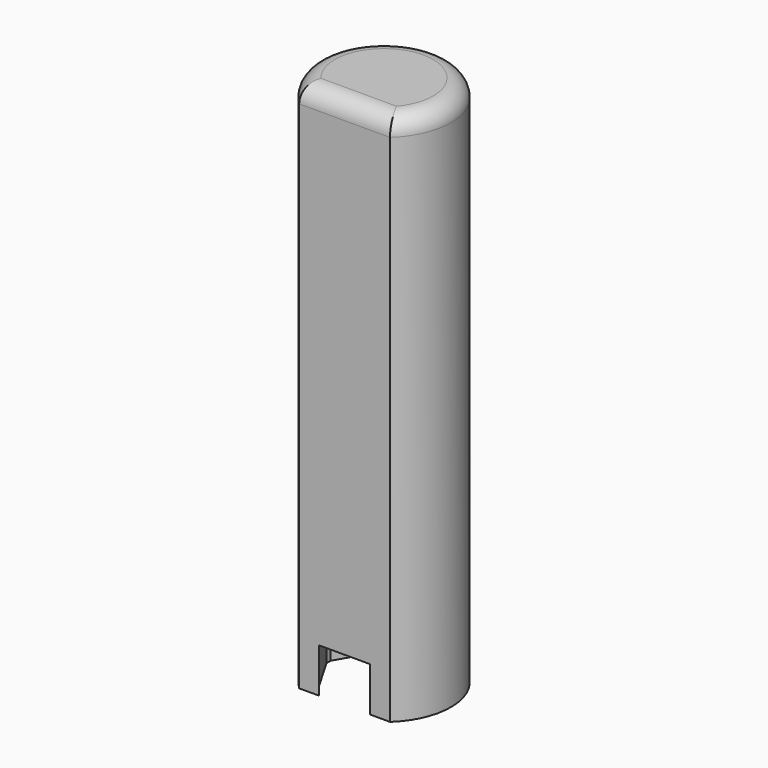
from build123d import *

# Parameters (mm, degrees)
F1_DEPTH    = 30
F2_DEPTH    = 2.5
F3_DEPTH    = 30
F4_T1_DEPTH = 10.1185935568
F4_T4_ANGLE = 350.8041938213


# Not quite as in the source:
# - a fillet or chamfer that OpenCascade refuses, or shapes differently, is made with other operations: its cross-section is extruded or revolved along the edge and cut away or added


with BuildPart() as f1:
    # F0 (on Top) → F1 (new body)
    with BuildSketch(Plane.XY):
        with BuildLine():
            Line((-1.4370107863, -2.775), (-1.602146997, -2.775))
            Line((-1.602146997, -2.775), (-2.5592967784, -2.775))
            ThreePointArc((-2.5592967784, -2.775), (0, -3.775), (2.5592967784, -2.775))
            Line((2.5592967784, -2.775), (1.602146997, -2.775))
            Line((1.602146997, -2.775), (1.4370107863, -2.775))
            ThreePointArc((1.4370107863, -2.775), (0, -3.125), (-1.4370107863, -2.775))
        make_face()
        with BuildLine():
            Line((-1.6847151023, 2.6319878465), (-1.602146997, 2.775))
            Line((-1.602146997, 2.775), (-1.4370107863, 2.775))
            ThreePointArc((-1.4370107863, 2.775), (0, 3.125), (1.4370107863, 2.775))
            Line((1.4370107863, 2.775), (1.602146997, 2.775))
            Line((1.602146997, 2.775), (1.6847151023, 2.6319878465))
            ThreePointArc((1.6847151023, 2.6319878465), (2.7063293868, 1.5625), (3.1217258887, 0.1430121535))
            Line((3.1217258887, 0.1430121535), (3.204293994, 0))
            Line((3.204293994, 0), (3.1217258887, -0.1430121535))
            ThreePointArc((3.1217258887, -0.1430121535), (2.7063293868, -1.5625), (1.6847151023, -2.6319878465))
            Line((1.6847151023, -2.6319878465), (1.602146997, -2.775))
            Line((1.602146997, -2.775), (2.5592967784, -2.775))
            ThreePointArc((2.5592967784, -2.775), (3.4577427853, -1.5148068625), (3.775, 0))
            ThreePointArc((3.775, 0), (-1.5148068625, 3.4577427853), (-2.5592967784, -2.775))
            Line((-2.5592967784, -2.775), (-1.602146997, -2.775))
            Line((-1.602146997, -2.775), (-1.6847151023, -2.6319878465))
            ThreePointArc((-1.6847151023, -2.6319878465), (-2.7063293868, -1.5625), (-3.1217258887, -0.1430121535))
            Line((-3.1217258887, -0.1430121535), (-3.204293994, 0))
            Line((-3.204293994, 0), (-3.1217258887, 0.1430121535))
            ThreePointArc((-3.1217258887, 0.1430121535), (-2.7063293868, 1.5625), (-1.6847151023, 2.6319878465))
        make_face()
        with BuildLine():
            ThreePointArc((3.1217258887, 0.1430121535), (2.7063293868, 1.5625), (1.6847151023, 2.6319878465))
            Line((1.6847151023, 2.6319878465), (3.1217258887, 0.1430121535))
        make_face()
        with BuildLine():
            Line((1.4370107863, -2.775), (-1.4370107863, -2.775))
            ThreePointArc((-1.4370107863, -2.775), (0, -3.125), (1.4370107863, -2.775))
        make_face()
        with BuildLine():
            ThreePointArc((1.4370107863, 2.775), (0, 3.125), (-1.4370107863, 2.775))
            Line((-1.4370107863, 2.775), (1.4370107863, 2.775))
        make_face()
        with BuildLine():
            Line((-3.1217258887, 0.1430121535), (-1.6847151023, 2.6319878465))
            ThreePointArc((-1.6847151023, 2.6319878465), (-2.7063293868, 1.5625), (-3.1217258887, 0.1430121535))
        make_face()
        with BuildLine():
            Line((1.4370107863, 2.775), (-1.4370107863, 2.775))
            ThreePointArc((-1.4370107863, 2.775), (-1.5625, 2.7063293868), (-1.6847151023, 2.6319878465))
            Line((-1.6847151023, 2.6319878465), (-3.1217258887, 0.1430121535))
            ThreePointArc((-3.1217258887, 0.1430121535), (-3.125, 0), (-3.1217258887, -0.1430121535))
            Line((-3.1217258887, -0.1430121535), (-1.6847151023, -2.6319878465))
            ThreePointArc((-1.6847151023, -2.6319878465), (-1.5625, -2.7063293868), (-1.4370107863, -2.775))
            Line((-1.4370107863, -2.775), (1.4370107863, -2.775))
            ThreePointArc((1.4370107863, -2.775), (1.5625, -2.7063293868), (1.6847151023, -2.6319878465))
            Line((1.6847151023, -2.6319878465), (3.1217258887, -0.1430121535))
            ThreePointArc((3.1217258887, -0.1430121535), (3.1241813649, -0.0715248136), (3.125, 0))
            ThreePointArc((3.125, 0), (3.1241813649, 0.0715248136), (3.1217258887, 0.1430121535))
            Line((3.1217258887, 0.1430121535), (1.6847151023, 2.6319878465))
            ThreePointArc((1.6847151023, 2.6319878465), (1.5625, 2.7063293868), (1.4370107863, 2.775))
        make_face()
        with BuildLine():
            Line((-1.6847151023, -2.6319878465), (-3.1217258887, -0.1430121535))
            ThreePointArc((-3.1217258887, -0.1430121535), (-2.7063293868, -1.5625), (-1.6847151023, -2.6319878465))
        make_face()
        with BuildLine():
            ThreePointArc((1.6847151023, -2.6319878465), (2.7063293868, -1.5625), (3.1217258887, -0.1430121535))
            Line((3.1217258887, -0.1430121535), (1.6847151023, -2.6319878465))
        make_face()
        with BuildLine():
            ThreePointArc((-1.4370107863, -2.775), (-1.5625, -2.7063293868), (-1.6847151023, -2.6319878465))
            Line((-1.6847151023, -2.6319878465), (-1.602146997, -2.775))
            Line((-1.602146997, -2.775), (-1.4370107863, -2.775))
        make_face()
        with BuildLine():
            ThreePointArc((1.6847151023, -2.6319878465), (1.5625, -2.7063293868), (1.4370107863, -2.775))
            Line((1.4370107863, -2.775), (1.602146997, -2.775))
            Line((1.602146997, -2.775), (1.6847151023, -2.6319878465))
        make_face()
        with BuildLine():
            Line((3.204293994, 0), (3.1217258887, 0.1430121535))
            ThreePointArc((3.1217258887, 0.1430121535), (3.1241813649, 0.0715248136), (3.125, 0))
            ThreePointArc((3.125, 0), (3.1241813649, -0.0715248136), (3.1217258887, -0.1430121535))
            Line((3.1217258887, -0.1430121535), (3.204293994, 0))
        make_face()
        with BuildLine():
            ThreePointArc((-3.1217258887, -0.1430121535), (-3.125, 0), (-3.1217258887, 0.1430121535))
            Line((-3.1217258887, 0.1430121535), (-3.204293994, 0))
            Line((-3.204293994, 0), (-3.1217258887, -0.1430121535))
        make_face()
        with BuildLine():
            Line((1.602146997, 2.775), (1.4370107863, 2.775))
            ThreePointArc((1.4370107863, 2.775), (1.5625, 2.7063293868), (1.6847151023, 2.6319878465))
            Line((1.6847151023, 2.6319878465), (1.602146997, 2.775))
        make_face()
        with BuildLine():
            Line((-1.4370107863, 2.775), (-1.602146997, 2.775))
            Line((-1.602146997, 2.775), (-1.6847151023, 2.6319878465))
            ThreePointArc((-1.6847151023, 2.6319878465), (-1.5625, 2.7063293868), (-1.4370107863, 2.775))
        make_face()
    extrude(amount=F1_DEPTH)

    # F0 (on Top) → F2 (cut)
    with BuildSketch(Plane.XY):
        with BuildLine():
            Line((1.4370107863, 2.775), (-1.4370107863, 2.775))
            ThreePointArc((-1.4370107863, 2.775), (-1.5625, 2.7063293868), (-1.6847151023, 2.6319878465))
            Line((-1.6847151023, 2.6319878465), (-3.1217258887, 0.1430121535))
            ThreePointArc((-3.1217258887, 0.1430121535), (-3.125, 0), (-3.1217258887, -0.1430121535))
            Line((-3.1217258887, -0.1430121535), (-1.6847151023, -2.6319878465))
            ThreePointArc((-1.6847151023, -2.6319878465), (-1.5625, -2.7063293868), (-1.4370107863, -2.775))
            Line((-1.4370107863, -2.775), (1.4370107863, -2.775))
            ThreePointArc((1.4370107863, -2.775), (1.5625, -2.7063293868), (1.6847151023, -2.6319878465))
            Line((1.6847151023, -2.6319878465), (3.1217258887, -0.1430121535))
            ThreePointArc((3.1217258887, -0.1430121535), (3.1241813649, -0.0715248136), (3.125, 0))
            ThreePointArc((3.125, 0), (3.1241813649, 0.0715248136), (3.1217258887, 0.1430121535))
            Line((3.1217258887, 0.1430121535), (1.6847151023, 2.6319878465))
            ThreePointArc((1.6847151023, 2.6319878465), (1.5625, 2.7063293868), (1.4370107863, 2.775))
        make_face()
    extrude(amount=F2_DEPTH, mode=Mode.SUBTRACT)

    # F0 (on Top) → F3 (cut, through all)
    with BuildSketch(Plane.XY):
        with BuildLine():
            Line((1.4370107863, -2.775), (-1.4370107863, -2.775))
            ThreePointArc((-1.4370107863, -2.775), (0, -3.125), (1.4370107863, -2.775))
        make_face()
        with BuildLine():
            Line((-1.4370107863, -2.775), (-1.602146997, -2.775))
            Line((-1.602146997, -2.775), (-2.5592967784, -2.775))
            ThreePointArc((-2.5592967784, -2.775), (0, -3.775), (2.5592967784, -2.775))
            Line((2.5592967784, -2.775), (1.602146997, -2.775))
            Line((1.602146997, -2.775), (1.4370107863, -2.775))
            ThreePointArc((1.4370107863, -2.775), (0, -3.125), (-1.4370107863, -2.775))
        make_face()
    extrude(amount=F3_DEPTH, mode=Mode.SUBTRACT)

    # F4: fillet of radius 1 on 2 edges, made by hand

    # F4_s2 → F4_t1 (cut)
    with BuildSketch(Plane.YZ.offset(-5.0592967784)):
        with BuildLine():
            ThreePointArc((-2.775, 29), (-2.4821067812, 29.7071067812), (-1.775, 30))
            Line((-1.775, 30), (-2.775, 30))
            Line((-2.775, 30), (-2.775, 29))
        make_face()
    extrude(amount=F4_T1_DEPTH, mode=Mode.SUBTRACT)

    # F4_s3 → F4_t4 (revolve, cut)
    with BuildSketch(Plane(origin=(0, 0, 0), x_dir=(0, 0, 1), z_dir=(-0.9967818129, -0.0801624442, 0))):
        with BuildLine():
            ThreePointArc((29, -3.775), (29.7071067812, -3.4821067812), (30, -2.775))
            Line((30, -2.775), (30, -3.775))
            Line((30, -3.775), (29, -3.775))
        make_face()
    revolve(axis=Axis((0, 0, 30), (0, 0, 1)), revolution_arc=F4_T4_ANGLE, mode=Mode.SUBTRACT)


solid = f1.part
